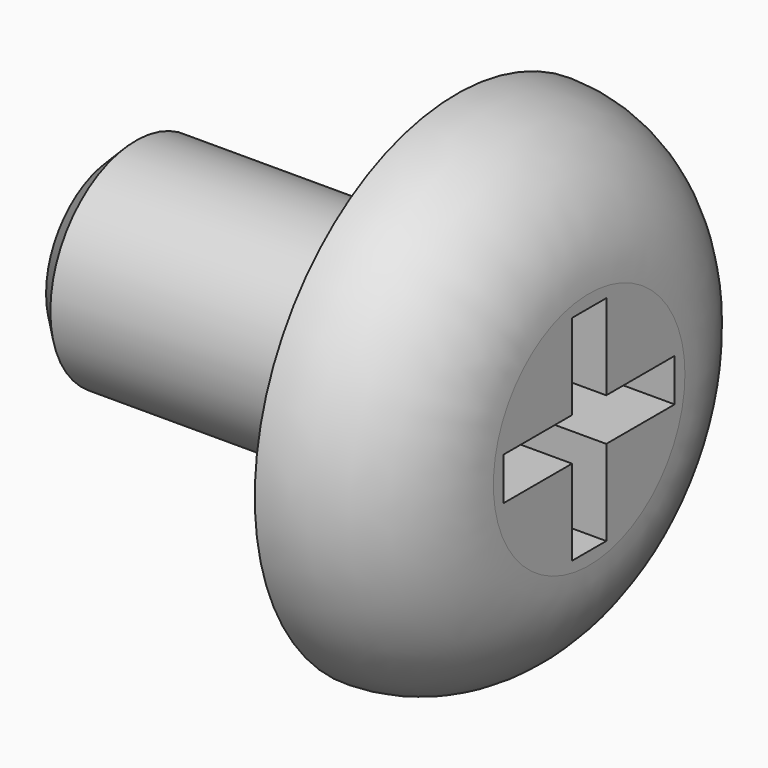
from build123d import *

# Parameters (mm, degrees)
F0_R     = 5.9
F1_DEPTH = 3.1
F2_R     = 3.09999
F4_DEPTH = 2
F5_R     = 2.5
F6_DEPTH = 8
F7_SIZE  = 0.5


# Not quite as in the source:
# - a fillet or chamfer is up to 0.001 mm smaller than in the source, because OpenCascade refuses the exact size


with BuildPart() as f1:
    # F0 (on Right) → F1 (new body)
    with BuildSketch(Plane.YZ):
        Circle(F0_R)
    extrude(amount=-F1_DEPTH)

    # F2 (radius 3.1 in the source; OpenCascade refuses exactly that, so slightly less here)
    f2_edges = [f1.edges().sort_by_distance(p)[0] for p in [
        (0, -5.9, 0),
    ]]
    fillet(f2_edges, radius=F2_R)

    # F3 (on face) → F4 (cut)
    with BuildSketch(Plane.YZ):
        Polygon((0.5, 2.5), (0, 2.5), (-0.5, 2.5), (-0.5, 0.5), (-2.5, 0.5), (-2.5, 0), (-2.5, -0.5), (-0.5, -0.5), (-0.5, -2.5), (0, -2.5), (0.5, -2.5), (0.5, -0.5), (2.5, -0.5), (2.5, 0), (2.5, 0.5), (0.5, 0.5), align=None)
    extrude(amount=-F4_DEPTH, mode=Mode.SUBTRACT)

    # F5 (on face) → F6 (join)
    with BuildSketch(Plane(origin=(-3.1, 0, 0), x_dir=(0, -1, 0), z_dir=(-1, 0, 0))):
        Circle(F5_R)
    extrude(amount=F6_DEPTH)

    # F7
    f7_edges = [f1.edges().sort_by_distance(p)[0] for p in [
        (-11.1, 2.5, 0),
    ]]
    chamfer(f7_edges, length=F7_SIZE)


solid = f1.part
